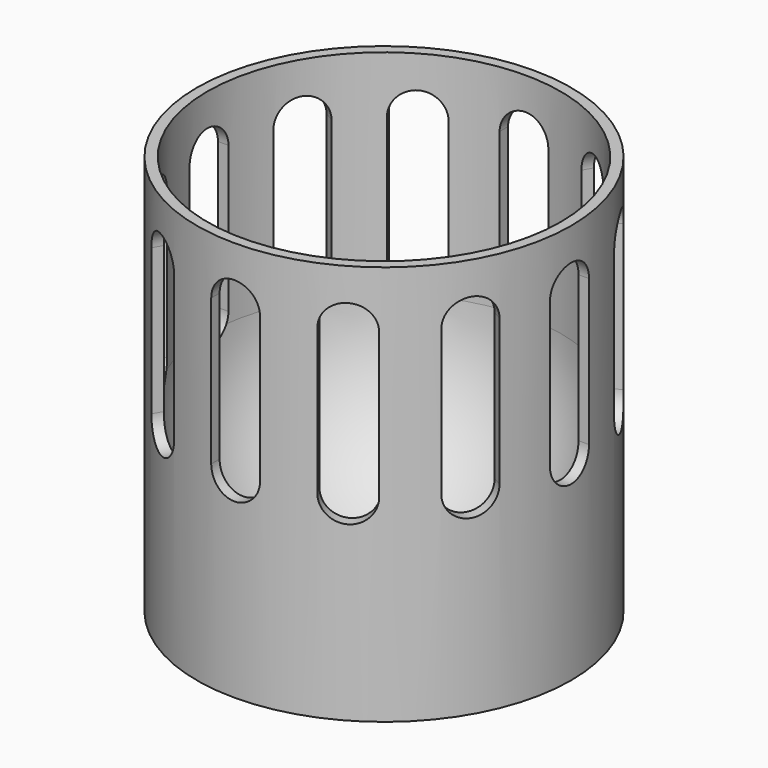
from build123d import *

# Parameters (mm, degrees)
F3_DEPTH        = 36.577
F3_COPIES_COUNT = 12


# Not quite as in the source:
# - a pattern or mirror of a feature is missing from the dataset's text; its kind, count and spacing are read off the source's solid


with BuildPart() as f1:
    # F0 (on Front) → F1 (revolve)
    with BuildSketch(Plane.XZ):
        with BuildLine():
            Line((36.576, 78.232), (34.544, 78.232))
            Line((34.544, 78.232), (34.544, 36.576))
            ThreePointArc((34.544, 36.576), (24.4262966493, 12.1497033507), (0, 2.032))
            Line((0, 2.032), (0, 0))
            Line((0, 0), (36.576, 0))
            Line((36.576, 0), (36.576, 78.232))
        make_face()
    revolve(axis=Axis((0, 0, 1.016), (0, 0, 1)))

    # F2 (on Front) → F3 (cut, through all)
    with BuildSketch(Plane.XZ):
        with BuildLine():
            Line((-4.7625, 67.1195), (-4.7625, 38.5445))
            ThreePointArc((-4.7625, 38.5445), (0, 33.782), (4.7625, 38.5445))
            Line((4.7625, 38.5445), (4.7625, 67.1195))
            ThreePointArc((4.7625, 67.1195), (0, 71.882), (-4.7625, 67.1195))
        make_face()
    f3 = extrude(amount=-F3_DEPTH, mode=Mode.SUBTRACT)

    # F3_copies: F3 ×12 about axis
    f3_copies_axis = Axis((0, 0, 0), (0, 0, 1))
    for i in range(1, F3_COPIES_COUNT):
        add(f3.rotate(f3_copies_axis, i * 360 / F3_COPIES_COUNT), mode=Mode.SUBTRACT)


solid = f1.part
